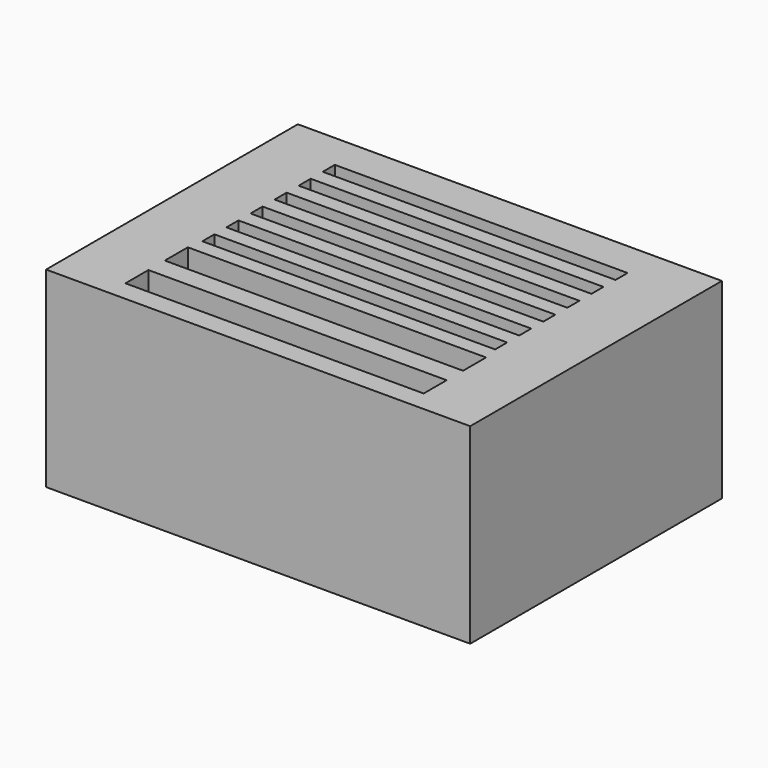
from build123d import *

# Parameters (mm, degrees)
F0_W     = 620
F0_H     = 460
F0_W_2   = 428
F0_H_2   = 22
F0_W_3   = 436
F0_H_3   = 42
F1_DEPTH = 280
F2_DEPTH = 250
F3_DEPTH = 140


# Not quite as in the source:
# - a feature names something its author has since deleted; it is built from what else it names


with BuildPart() as f1:
    # F0 (on Top) → F1 (new body)
    with BuildSketch(Plane.XY):
        with Locations((0.344911406, 64)):
            Rectangle(F0_W, F0_H)
        with Locations((0, 11)):
            Rectangle(F0_W_2, F0_H_2, mode=Mode.SUBTRACT)
        with Locations((0, 55)):
            Rectangle(F0_W_2, F0_H_2, mode=Mode.SUBTRACT)
        with Locations((0.344911406, -115)):
            Rectangle(F0_W_3, F0_H_3, mode=Mode.SUBTRACT)
        with Locations((0.344911406, -43)):
            Rectangle(F0_W_3, F0_H_3, mode=Mode.SUBTRACT)
        with Locations((0, 99)):
            Rectangle(F0_W_2, F0_H_2, mode=Mode.SUBTRACT)
        with Locations((0, 143)):
            Rectangle(F0_W_2, F0_H_2, mode=Mode.SUBTRACT)
        with Locations((0, 187)):
            Rectangle(F0_W_2, F0_H_2, mode=Mode.SUBTRACT)
        with Locations((0, 231)):
            Rectangle(F0_W_2, F0_H_2, mode=Mode.SUBTRACT)
        with Locations((0.344911406, -43)):
            Rectangle(F0_W_3, F0_H_3)
        with Locations((0.344911406, -115)):
            Rectangle(F0_W_3, F0_H_3)
        with Locations((0, 11)):
            Rectangle(F0_W_2, F0_H_2)
        with Locations((0, 55)):
            Rectangle(F0_W_2, F0_H_2)
        with Locations((0, 99)):
            Rectangle(F0_W_2, F0_H_2)
        with Locations((0, 143)):
            Rectangle(F0_W_2, F0_H_2)
        with Locations((0, 187)):
            Rectangle(F0_W_2, F0_H_2)
        with Locations((0, 231)):
            Rectangle(F0_W_2, F0_H_2)
    extrude(amount=-F1_DEPTH)

    # F0 (on Top) → F2 (cut)
    with BuildSketch(Plane.XY):
        with Locations((0.344911406, -43)):
            Rectangle(F0_W_3, F0_H_3)
        with Locations((0.344911406, -115)):
            Rectangle(F0_W_3, F0_H_3)
    extrude(amount=-F2_DEPTH, mode=Mode.SUBTRACT)

    # F0 (on Top) → F3 (cut)
    with BuildSketch(Plane.XY):
        with Locations((0, 11)):
            Rectangle(F0_W_2, F0_H_2)
        with Locations((0, 55)):
            Rectangle(F0_W_2, F0_H_2)
        with Locations((0, 99)):
            Rectangle(F0_W_2, F0_H_2)
        with Locations((0, 143)):
            Rectangle(F0_W_2, F0_H_2)
        with Locations((0, 187)):
            Rectangle(F0_W_2, F0_H_2)
        with Locations((0, 231)):
            Rectangle(F0_W_2, F0_H_2)
    extrude(amount=-F3_DEPTH, mode=Mode.SUBTRACT)


solid = f1.part
